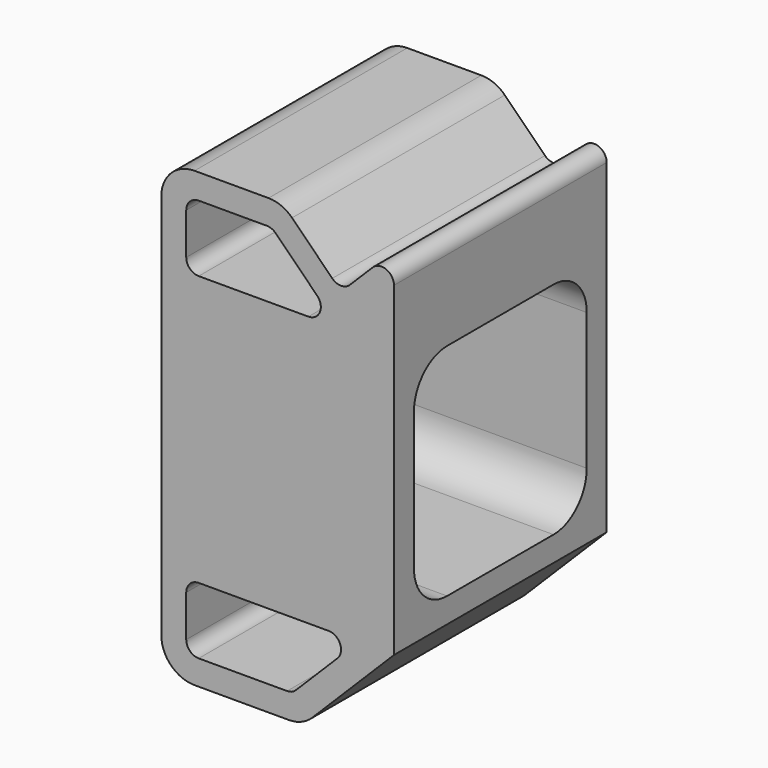
from build123d import *

# Parameters (mm, degrees)
F0_W          = 32
F0_H          = 32.5
F0_W_2        = 26
F0_H_2        = 26.5
F1_DEPTH      = 28
F3_DEPTH      = 16
F5_DEPTH      = 16
F5_DEPTH_BACK = 16
F6_R          = 5
F7_R          = 1.5
F8_R          = 4


# Not quite as in the source:
# - a feature names something its author has since deleted; it is built from what else it names


with BuildPart() as f1:
    # F0 (on Right) → F1 (new body)
    with BuildSketch(Plane.YZ):
        Rectangle(F0_W, F0_H)
        Rectangle(F0_W_2, F0_H_2, mode=Mode.SUBTRACT)
    extrude(amount=F1_DEPTH)

    # F2 (on Front) → F3 (join, symmetric)
    with BuildSketch(Plane.XZ):
        Polygon((21.3223304703, 16.25), (28, 16.25), (28, 26.5428932188), (21.6360389693, 20.1789321881), (14.5649711575, 27.25), (0, 27.25), (0, 16.25), (3, 16.25), (3, 24.25), (13.3223304703, 24.25), align=None)
    extrude(amount=F3_DEPTH, both=True)

    # F4 (on Front) → F5 (join, two sides)
    with BuildSketch(Plane.XZ) as f5_sk:
        Polygon((3, -16.25), (0, -16.25), (0, -27.25), (17, -27.25), (28, -16.25), (23.7573593129, -16.25), (15.7573593129, -24.25), (3, -24.25), align=None)
    extrude(amount=F5_DEPTH)
    extrude(f5_sk.sketch, amount=-F5_DEPTH_BACK)

    # F6
    f6_edges = [f1.edges().sort_by_distance(p)[0] for p in [
        (14, 13, -13.25),
        (14, 13, 13.25),
        (14, -13, 13.25),
        (14, -13, -13.25),
    ]]
    fillet(f6_edges, radius=F6_R)

    # F7
    f7_edges = [f1.edges().sort_by_distance(p)[0] for p in [
        (3, 0, 16.25),
        (3, 0, 24.25),
        (13.32233, 0, 24.25),
        (21.32233, 0, 16.25),
        (21.636039, 0, 20.178932),
        (28, 0, 26.542893),
        (3, 0, -16.25),
        (23.757359, 0, -16.25),
        (15.757359, 0, -24.25),
        (3, 0, -24.25),
    ]]
    fillet(f7_edges, radius=F7_R)

    # F8
    f8_edges = [f1.edges().sort_by_distance(p)[0] for p in [
        (0, 0, 27.25),
        (14.564971, 0, 27.25),
        (0, 0, -27.25),
        (17, 0, -27.25),
    ]]
    fillet(f8_edges, radius=F8_R)


solid = f1.part
